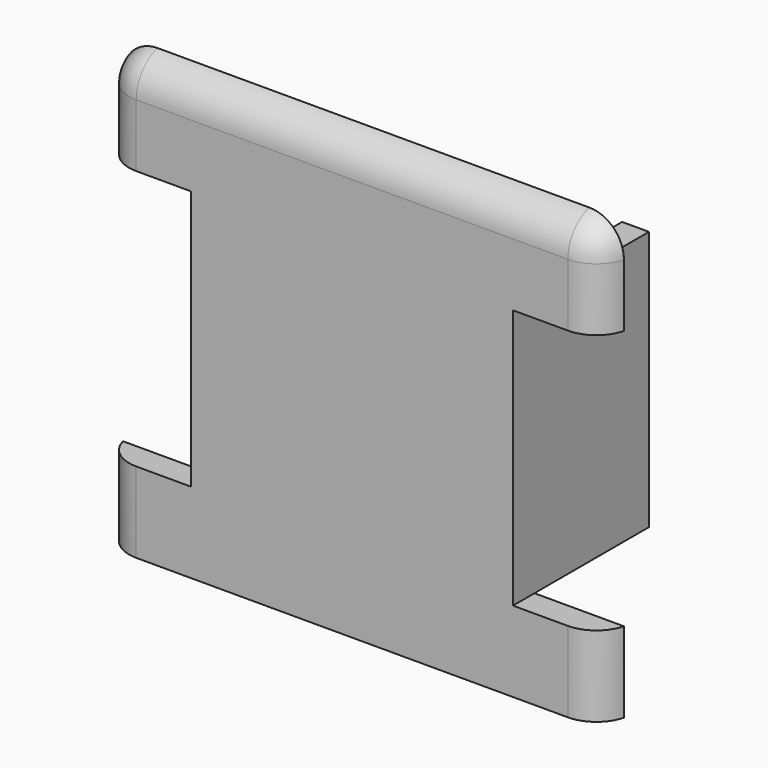
from build123d import *

# Parameters (mm, degrees)
F1_DEPTH    = 12.271
F2_T1_DEPTH = 12.0635083269
F2_T4_ANGLE = 218.8024505591
F2_T6_ANGLE = 218.8024505591
F3_W        = 2.5
F3_H        = 7.2664258366
F4_DEPTH    = 0.751
F5_W        = 0.75
F5_H        = 7.2664258366
F6_DEPTH    = 4


# Not quite as in the source:
# - a fillet or chamfer that OpenCascade refuses, or shapes differently, is made with other operations: its cross-section is extruded or revolved along the edge and cut away or added


with BuildPart() as f1:
    # F0 (on Top) → F1 (new body)
    with BuildSketch(Plane.XY):
        with BuildLine():
            Line((1.5818497799, 3.6993569562), (-12.4181502201, 3.6993569562))
            ThreePointArc((-12.4181502201, 3.6993569562), (-12.0622768192, 3.1587875411), (-11.4499043835, 2.9493569562))
            Line((-11.4499043835, 2.9493569562), (0.6136039434, 2.9493569562))
            ThreePointArc((0.6136039434, 2.9493569562), (1.2259763791, 3.1587875411), (1.5818497799, 3.6993569562))
        make_face()
    extrude(amount=F1_DEPTH)

    # F2: fillet of radius 1 on 1 edges, made by hand

    # F2_s2 → F2_t1 (cut)
    with BuildSketch(Plane.YZ.offset(-11.4499043835)):
        with BuildLine():
            ThreePointArc((2.9493569562, 11.271), (3.242250175, 11.9781067812), (3.9493569562, 12.271))
            Line((3.9493569562, 12.271), (2.9493569562, 12.271))
            Line((2.9493569562, 12.271), (2.9493569562, 11.271))
        make_face()
    extrude(amount=F2_T1_DEPTH, mode=Mode.SUBTRACT)

    # F2_s3 → F2_t4 (revolve, cut)
    with BuildSketch(Plane(origin=(-8.8824733702, 7.1423174648, 0), x_dir=(0, 0, 1), z_dir=(0.7793111642, -0.6266371433, 0))):
        with BuildLine():
            ThreePointArc((11.271, 3.0971574071), (11.9781067812, 3.3900506259), (12.271, 4.0971574071))
            Line((12.271, 4.0971574071), (12.271, 3.0971574071))
            Line((12.271, 3.0971574071), (11.271, 3.0971574071))
        make_face()
    revolve(axis=Axis((-11.4499043835, 3.9493569562, 12.271), (0, 0, 1)), revolution_arc=F2_T4_ANGLE, mode=Mode.SUBTRACT)

    # F2_s5 → F2_t6 (revolve, cut)
    with BuildSketch(Plane.YZ.offset(0.6136039434)):
        with BuildLine():
            ThreePointArc((2.9493569562, 11.271), (3.242250175, 11.9781067812), (3.9493569562, 12.271))
            Line((3.9493569562, 12.271), (2.9493569562, 12.271))
            Line((2.9493569562, 12.271), (2.9493569562, 11.271))
        make_face()
    revolve(axis=Axis((0.6136039434, 3.9493569562, 12.271), (0, 0, 1)), revolution_arc=F2_T6_ANGLE, mode=Mode.SUBTRACT)

    # F3 (on face) → F4 (cut, through all)
    with BuildSketch(Plane(origin=(0, 3.6993569562, 0), x_dir=(-1, 0, 0), z_dir=(0, 1, 0))):
        with Locations((11.1681502201, 5.8831429183)):
            Rectangle(F3_W, F3_H)
        with Locations((-0.3318497799, 5.8831429183)):
            Rectangle(F3_W, F3_H)
    extrude(amount=-F4_DEPTH, mode=Mode.SUBTRACT)

    # F5 (on face) → F6 (join)
    with BuildSketch(Plane(origin=(0, 3.6993569562, 0), x_dir=(-1, 0, 0), z_dir=(0, 1, 0))):
        with Locations((1.2931502201, 5.8831429183)):
            Rectangle(F5_W, F5_H)
        with Locations((9.5431502201, 5.8831429183)):
            Rectangle(F5_W, F5_H)
    extrude(amount=F6_DEPTH)


solid = f1.part
